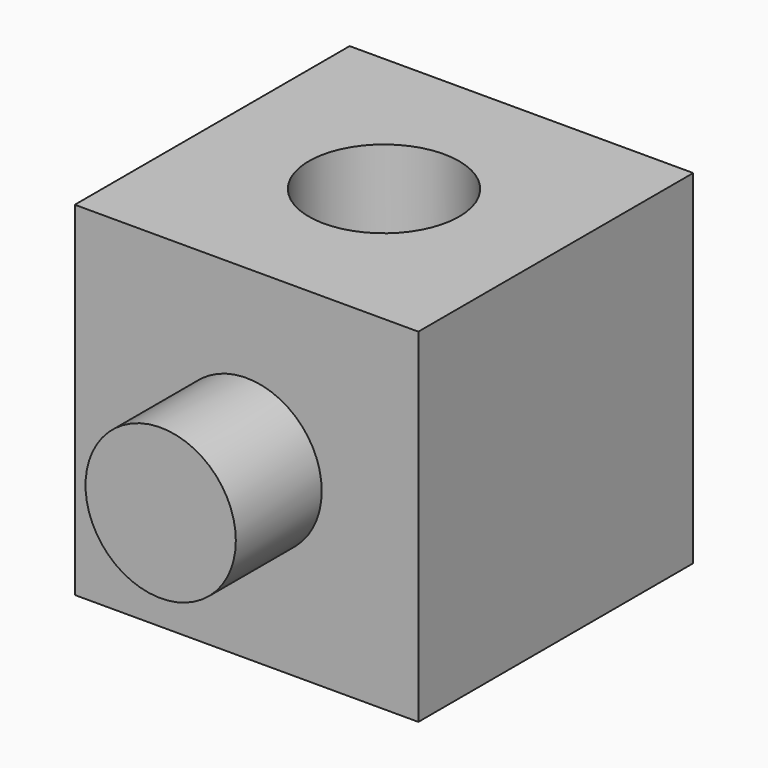
from build123d import *

# Parameters (mm, degrees)
F0_W     = 80
F0_H     = 80
F1_DEPTH = 80
F2_R     = 17.5
F3_DEPTH = 25
F4_R     = 17.5
F5_DEPTH = 80.001
F6_T     = -2.5


with BuildPart() as f1:
    # F0 (on Front) → F1 (new body)
    with BuildSketch(Plane.XZ):
        Rectangle(F0_W, F0_H)
    extrude(amount=F1_DEPTH)

    # F2 (on face) → F3 (join)
    with BuildSketch(Plane.XZ.offset(80)):
        Circle(F2_R)
    extrude(amount=F3_DEPTH)

    # F4 (on face) → F5 (cut, through all)
    with BuildSketch(Plane.XY.offset(40)):
        with Locations((0, -40)):
            Circle(F4_R)
    extrude(amount=-F5_DEPTH, mode=Mode.SUBTRACT)

    # F6
    f6_openings = [f1.faces().sort_by_distance(p)[0] for p in [
        (-38.868629, -40, -40),
    ]]
    offset(amount=F6_T, openings=f6_openings, kind=Kind.INTERSECTION)


solid = f1.part
